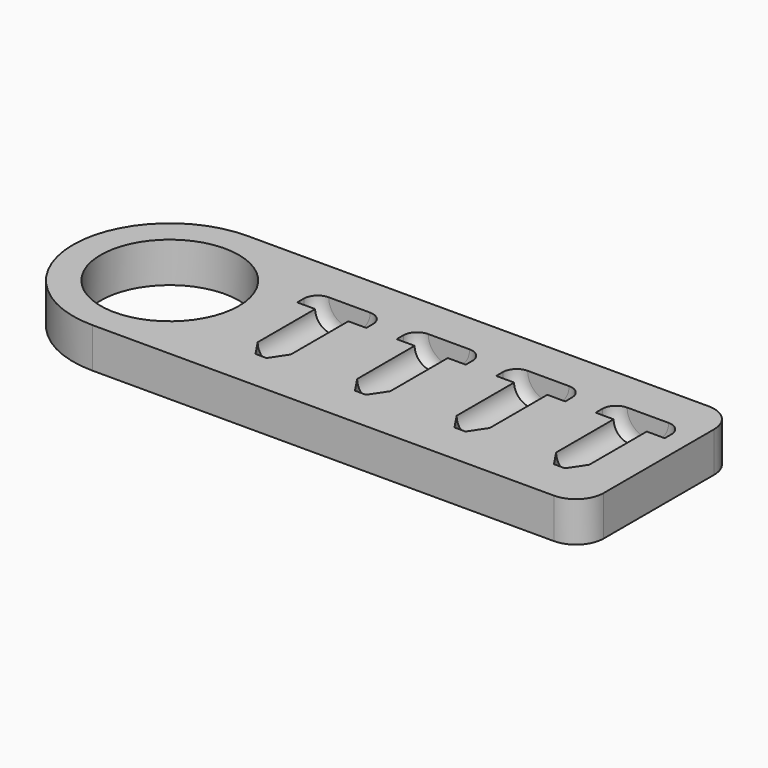
from build123d import *

# Parameters (mm, degrees)
F0_R         = 12.5
F1_DEPTH     = 7.25
F7_TEXT_SIZE = 5.5555555556
F8_DEPTH     = 1


# Not quite as in the source:
# - Text() gives the source's letters only with a copy of the font that has no kerning and outlines rounded to 1/6400 em; it was checked with that copy


with BuildPart() as f1:
    # F0 (on Top) → F1 (new body)
    with BuildSketch(Plane.XY):
        with BuildLine():
            ThreePointArc((0, 17.5), (5.1256313292, 5.1256313292), (17.5, 0))
            Line((17.5, 0), (101, 0))
            ThreePointArc((101, 0), (104.5355339059, 1.4644660941), (106, 5))
            Line((106, 5), (106, 30))
            ThreePointArc((106, 30), (104.5355339059, 33.5355339059), (101, 35))
            Line((101, 35), (17.5, 35))
            ThreePointArc((17.5, 35), (5.1256313292, 29.8743686708), (0, 17.5))
        make_face()
        with Locations((17.5, 17.5)):
            Circle(F0_R, mode=Mode.SUBTRACT)
    extrude(amount=F1_DEPTH)

    # F2 (on face) → F3 (revolve, cut)
    with BuildSketch(Plane.XY.offset(7.25)):
        with BuildLine():
            Line((42, 10.5), (42, 7.5))
            Line((42, 7.5), (43, 7.5))
            Line((43, 7.5), (45, 10.5))
            Line((45, 10.5), (45, 23.5))
            Line((45, 23.5), (48.25, 23.5))
            Line((48.25, 23.5), (48.25, 25))
            ThreePointArc((48.25, 25), (47.517766953, 26.767766953), (45.75, 27.5))
            Line((45.75, 27.5), (42, 27.5))
            Line((42, 27.5), (42, 23.5))
            Line((42, 23.5), (42, 10.5))
        make_face()
    revolve(axis=Axis((42, 15.5, 7.25), (0, 1, 0)), mode=Mode.SUBTRACT)

    # F2 (on face) → F4 (revolve, cut)
    with BuildSketch(Plane.XY.offset(7.25)):
        with BuildLine():
            Line((60, 10.5), (60, 7.5))
            Line((60, 7.5), (61, 7.5))
            Line((61, 7.5), (63, 10.5))
            Line((63, 10.5), (63, 23.5))
            Line((63, 23.5), (66.25, 23.5))
            Line((66.25, 23.5), (66.25, 25))
            ThreePointArc((66.25, 25), (65.517766953, 26.767766953), (63.75, 27.5))
            Line((63.75, 27.5), (60, 27.5))
            Line((60, 27.5), (60, 23.5))
            Line((60, 23.5), (60, 10.5))
        make_face()
    revolve(axis=Axis((60, 15.5, 7.25), (0, 1, 0)), mode=Mode.SUBTRACT)

    # F2 (on face) → F5 (revolve, cut)
    with BuildSketch(Plane.XY.offset(7.25)):
        with BuildLine():
            Line((78, 10.5), (78, 7.5))
            Line((78, 7.5), (79, 7.5))
            Line((79, 7.5), (81, 10.5))
            Line((81, 10.5), (81, 23.5))
            Line((81, 23.5), (84.25, 23.5))
            Line((84.25, 23.5), (84.25, 25))
            ThreePointArc((84.25, 25), (83.517766953, 26.767766953), (81.75, 27.5))
            Line((81.75, 27.5), (78, 27.5))
            Line((78, 27.5), (78, 23.5))
            Line((78, 23.5), (78, 10.5))
        make_face()
    revolve(axis=Axis((78, 17, 7.25), (0, -1, 0)), mode=Mode.SUBTRACT)

    # F2 (on face) → F6 (revolve, cut)
    with BuildSketch(Plane.XY.offset(7.25)):
        with BuildLine():
            Line((96, 10.5), (96, 7.5))
            Line((96, 7.5), (97, 7.5))
            Line((97, 7.5), (99, 10.5))
            Line((99, 10.5), (99, 23.5))
            Line((99, 23.5), (102.25, 23.5))
            Line((102.25, 23.5), (102.25, 25))
            ThreePointArc((102.25, 25), (101.517766953, 26.767766953), (99.75, 27.5))
            Line((99.75, 27.5), (96, 27.5))
            Line((96, 27.5), (96, 23.5))
            Line((96, 23.5), (96, 10.5))
        make_face()
    revolve(axis=Axis((96, 15.5, 7.25), (0, 1, 0)), mode=Mode.SUBTRACT)

    # F7 (on face) → F8 (cut)
    with BuildSketch(Plane(origin=(0, 0, 0), x_dir=(1, 0, 0), z_dir=(0, 0, -1))):
        with Locations((30, -9)):
            Text('950', F7_TEXT_SIZE, font='Open Sans', text_align=(TextAlign.LEFT, TextAlign.BOTTOM))
    extrude(amount=-F8_DEPTH, mode=Mode.SUBTRACT)


solid = f1.part
